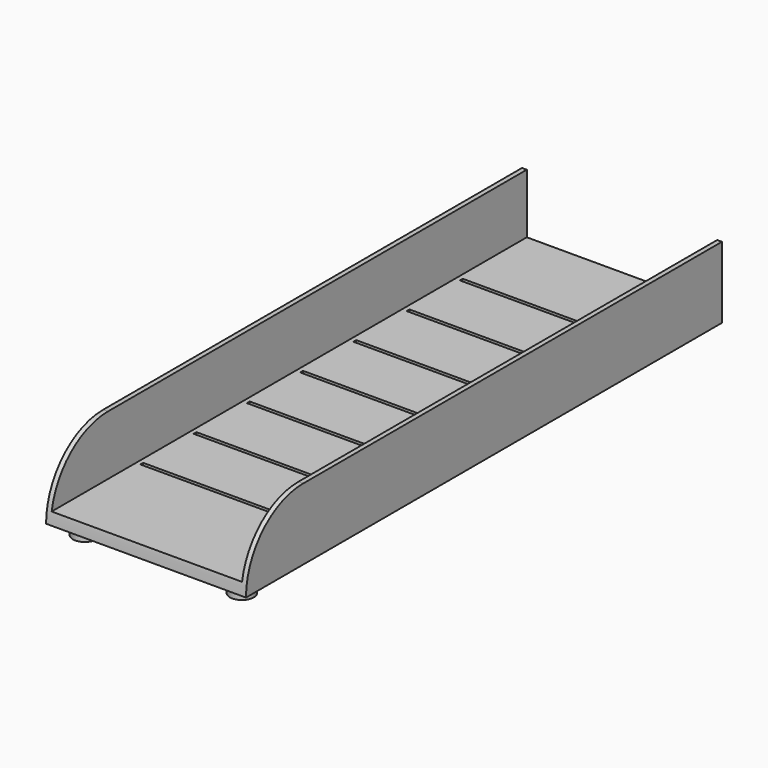
from build123d import *

# Parameters (mm, degrees)
F0_W     = 84
F0_H     = 30
F1_DEPTH = 250
F2_W     = 80
F2_H     = 50.6085516345
F3_DEPTH = 250.001
F4_R     = 5
F5_DEPTH = 5
F6_W     = 76
F6_H     = 1.5
F7_DEPTH = 25.4
F8_F1_R  = 29.9999


# Not quite as in the source:
# - a fillet or chamfer is up to 0.001 mm smaller than in the source, because OpenCascade refuses the exact size


with BuildPart() as f1:
    # F0 (on Front) → F1 (new body)
    with BuildSketch(Plane.XZ):
        with Locations((-42, 15)):
            Rectangle(F0_W, F0_H)
    extrude(amount=-F1_DEPTH)

    # F2 (on Front) → F3 (cut, through all)
    with BuildSketch(Plane.XZ):
        with Locations((-42, 30.3042758173)):
            Rectangle(F2_W, F2_H)
    extrude(amount=-F3_DEPTH, mode=Mode.SUBTRACT)

    # F4 (on face) → F5 (join)
    with BuildSketch(Plane(origin=(0, 0, 0), x_dir=(1, 0, 0), z_dir=(0, 0, -1))):
        with Locations((-75.0694796443, -9.1842794791)):
            Circle(F4_R)
        with Locations((-9.0694796443, -9.1842794791)):
            Circle(F4_R)
        with BuildLine():
            add(Edge.make_bspline(
                [(-42, -228.9691147673), (-42, -236.5294238205), (-42, -242.7407619737), (-42, -247.3817589414)],
                knots=[0.7062379003, 0.7062379003, 0.7062379003, 0.7062379003, 0.8221337183, 0.8221337183, 0.8221337183, 0.8221337183], degree=3))
            add(Edge.make_bspline(
                [(-42, -228.9691147673), (-72.1999239177, -228.6668722572), (-72.1999239177, -238.1754368544), (-72.1999239177, -247.6840014516), (-42, -247.3817589414)],
                knots=[1.5390046272, 1.5390046272, 1.5390046272, 3.1415926536, 3.1415926536, 4.74418068, 4.74418068, 4.74418068], degree=2, weights=[1, 0.695777858, 1, 0.695777858, 1]))
        make_face()
        with BuildLine():
            add(Edge.make_bspline(
                [(-42, -247.3817589414), (-13.660820201, -247.0981388613), (-13.660820201, -238.1754368544)],
                knots=[4.74418068, 4.74418068, 4.74418068, 6.2831853072, 6.2831853072, 6.2831853072], degree=2, weights=[1, 0.7182570377, 1]))
            add(Edge.make_bspline(
                [(-13.660820201, -238.1754368544), (-13.660820201, -229.2527348474), (-42, -228.9691147673)],
                knots=[0, 0, 0, 1.5390046272, 1.5390046272, 1.5390046272], degree=2, weights=[1, 0.7182570377, 1]))
            add(Edge.make_bspline(
                [(-42, -228.9691147673), (-42, -236.5294238205), (-42, -242.7407619737), (-42, -247.3817589414)],
                knots=[0.7062379003, 0.7062379003, 0.7062379003, 0.7062379003, 0.8221337183, 0.8221337183, 0.8221337183, 0.8221337183], degree=3))
        make_face()
    extrude(amount=F5_DEPTH)

    # F6 (on face) → F7 (cut)
    with BuildSketch(Plane.XY.offset(5)):
        with Locations((-42, 213.1024897098)):
            Rectangle(F6_W, F6_H)
        with Locations((-42.0274770269, 185.1625032207)):
            Rectangle(F6_W, F6_H)
        with Locations((-42.0549540537, 157.2225167316)):
            Rectangle(F6_W, F6_H)
        with Locations((-42.1648621612, 45.462570775)):
            Rectangle(F6_W, F6_H)
        with Locations((-42.1373851343, 73.4025572642)):
            Rectangle(F6_W, F6_H)
        with Locations((-42.1099081074, 101.3425437533)):
            Rectangle(F6_W, F6_H)
        with Locations((-42.0824310806, 129.2825302424)):
            Rectangle(F6_W, F6_H)
    extrude(amount=-F7_DEPTH, mode=Mode.SUBTRACT)

    # F8: fillet of radius 30 on 2 edges, made by hand

    # F8_f1 (radius 30 in the source; OpenCascade refuses exactly that, so slightly less here)
    f8_f1_edges = [f1.edges().sort_by_distance(p)[0] for p in [
        (-83, 0, 30),
    ]]
    fillet(f8_f1_edges, radius=F8_F1_R)


solid = f1.part
